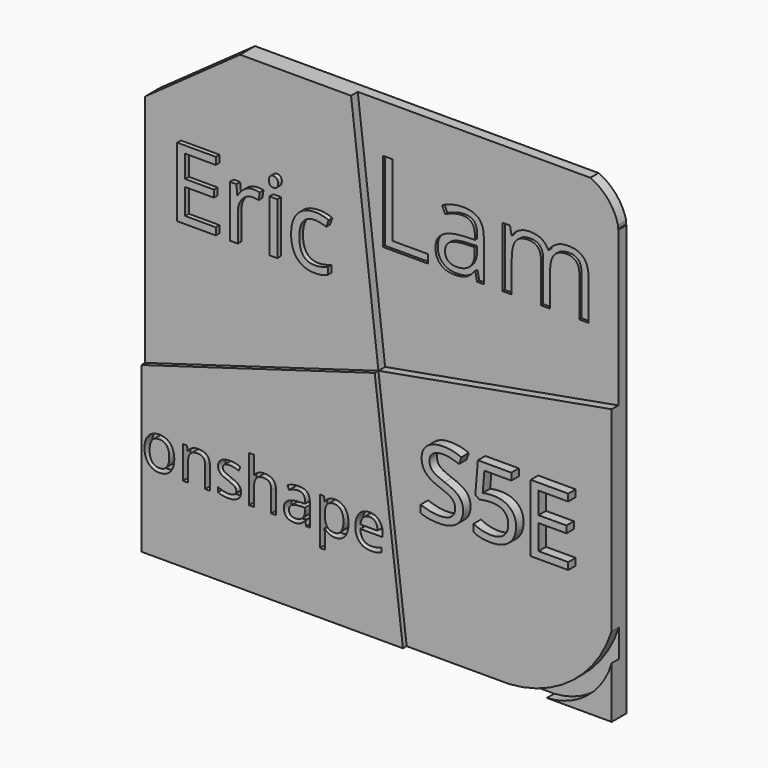
from build123d import *

# Parameters (mm, degrees)
F1_DEPTH      = 2
F3_DEPTH      = 0.9
F5_DEPTH      = 0.5
F6_TEXT_SIZE  = 10.3886278036
F7_DEPTH      = 0.5
F8_TEXT_SIZE  = 12.0653473358
F9_DEPTH      = 0.3
F10_TEXT_SIZE = 6.4966863849
F11_DEPTH     = 1
F12_TEXT_SIZE = 10.0981702821
F13_DEPTH     = 1
F15_DEPTH     = 25
F17_DEPTH     = 25
F19_DEPTH     = 1


# Not quite as in the source:
# - Text() gives the source's letters only with a copy of the font that has no kerning and outlines rounded to 1/6400 em; it was checked with that copy


with BuildPart() as f1:
    # F0 (on Front) → F1 (new body)
    with BuildSketch(Plane.XZ):
        Polygon((6.25, -25), (25, -25), (25, 25), (0, 25), (0, 0), align=None)
        Polygon((-6.252431527, -25), (6.25, -25), (0, 0), align=None)
        Polygon((-25, -25), (-6.252431527, -25), (0, 0), (0, 25), (-25, 25), align=None)
    extrude(amount=-F1_DEPTH)

    # F2 (on face) → F3 (cut)
    with BuildSketch(Plane.XZ):
        Polygon((-2.9271584935, 25), (0, 0), (25, 4.4977129437), (25, 25), align=None)
    extrude(amount=-F3_DEPTH, mode=Mode.SUBTRACT)

    # F4 (on face) → F5 (join)
    with BuildSketch(Plane.XZ):
        Polygon((3.0301702209, -25), (0, 0), (-25, -7.3816692457), (-25, -25), align=None)
    extrude(amount=F5_DEPTH)

    # F6 (on face) → F7 (join)
    with BuildSketch(Plane.XZ):
        with Locations((-22.1844855696, 7.4334405363)):
            Text('Eric', F6_TEXT_SIZE, font='Open Sans', text_align=(TextAlign.LEFT, TextAlign.BOTTOM))
    extrude(amount=F7_DEPTH)

    # F8 (on face) → F9 (cut)
    with BuildSketch(Plane.XZ.offset(-0.9)):
        with Locations((-1.4163665473, 11.2365102395)):
            Text('Lam', F8_TEXT_SIZE, font='Open Sans', text_align=(TextAlign.LEFT, TextAlign.BOTTOM))
    extrude(amount=-F9_DEPTH, mode=Mode.SUBTRACT)

    # F10 (on face) → F11 (cut)
    with BuildSketch(Plane.XZ.offset(0.5)):
        with Locations((-25.0330892159, -16.8593367562)):
            Text('onshape', F10_TEXT_SIZE, font='Open Sans', text_align=(TextAlign.LEFT, TextAlign.BOTTOM))
    extrude(amount=-F11_DEPTH, mode=Mode.SUBTRACT)

    # F12 (on face) → F13 (join)
    with BuildSketch(Plane.XZ):
        with Locations((4.8156478442, -11.519782478)):
            Text('S5E', F12_TEXT_SIZE, font='Open Sans', text_align=(TextAlign.LEFT, TextAlign.BOTTOM))
    extrude(amount=F13_DEPTH)

    # F14 (on face) → F15 (cut)
    with BuildSketch(Plane.XZ):
        Polygon((-25, 25), (-25, 17.7517980337), (-14.8246409371, 25), align=None)
    extrude(amount=-F15_DEPTH, mode=Mode.SUBTRACT)

    # F16 (on face) → F17 (cut)
    with BuildSketch(Plane.XZ.offset(-0.9)):
        with BuildLine():
            ThreePointArc((24.9564374952, 21.4975748833), (24.9480165452, 21.2991037198), (24.9307198637, 21.1012084445))
            Line((24.9307198637, 21.1012084445), (25, 21.0553500801))
            Line((25, 21.0553500801), (25, 25))
            Line((25, 25), (21.9943785501, 25))
            ThreePointArc((21.9943785501, 25), (23.8848898774, 23.59509303), (24.9564374952, 21.4975748833))
        make_face()
    extrude(amount=-F17_DEPTH, mode=Mode.SUBTRACT)

    # F18 (on face) → F19 (cut)
    with BuildSketch(Plane.XZ):
        with BuildLine():
            Line((14.0150851104, -25), (17.2041784972, -25))
            Line((17.2041784972, -25), (18.0500229004, -25))
            ThreePointArc((18.0500229004, -25), (22.4109527017, -23.3367127835), (25, -19.4532778114))
            Line((25, -19.4532778114), (25, -16.414353624))
            ThreePointArc((25, -16.414353624), (20.8393257127, -22.4111282671), (14.0150851104, -25))
        make_face()
    extrude(amount=-F19_DEPTH, mode=Mode.SUBTRACT)


solid = f1.part
